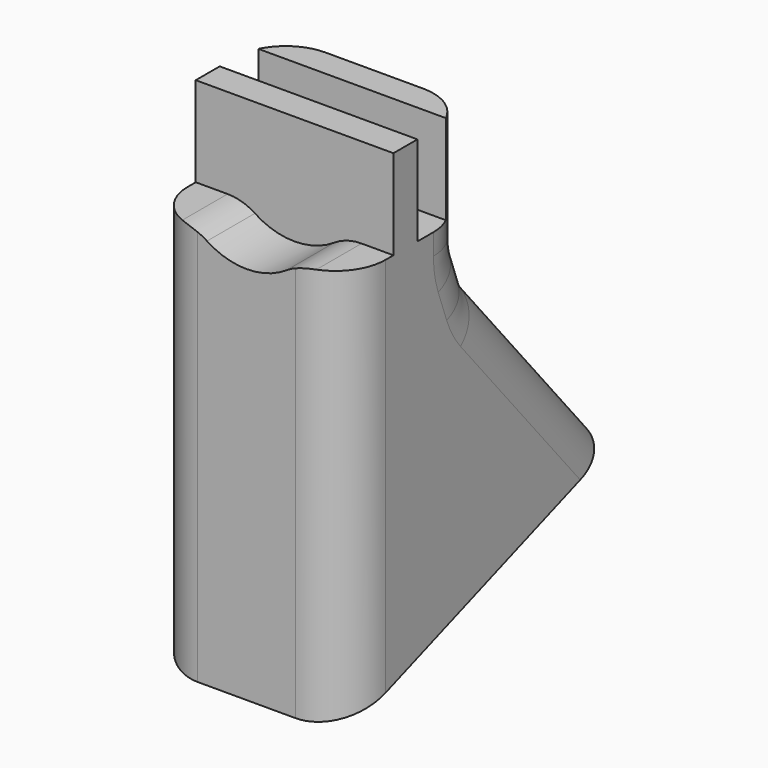
from build123d import *

# Parameters (mm, degrees)
F0_W     = 2.8
F0_H     = 9
F1_DEPTH = 19.8
F3_F1_R  = 5
F3_F2_R  = 5
F4_DEPTH = 6
F5_R     = 5


# Not quite as in the source:
# - a feature of the source that left no trace in its solid (it failed there, or was rolled back) is left out


with BuildPart() as f1:
    # F0 (on Right) → F1 (new body)
    with BuildSketch(Plane.YZ):
        Polygon((0, 9), (0, 0), (3, 0), (3, 2.7590821834), (3, 9), align=None)
        with Locations((8.6, 4.5)):
            Rectangle(F0_W, F0_H)
        Polygon((3, 0), (0, 0), (0, -3), (7.832443736, -3), (5.3151448425, 0), align=None)
        Polygon((7.2, 0), (5.3151448425, 0), (7.832443736, -3), (10, -3), (10, 0), align=None)
        Polygon((0, -3), (0, 0), (-6, 0), (-6, -40), (20.0199263242, -30.5295213202), (11.6604444312, -7.562033581), (7.832443736, -3), align=None)
        Polygon((10, -3), (7.832443736, -3), (11.6604444312, -7.562033581), align=None)
        Polygon((28.3794082171, -27.4869187373), (11.6604444312, -7.562033581), (20.0199263242, -30.5295213202), align=None)
    extrude(amount=F1_DEPTH)

    # F3: fillet of radius 5 on 6 edges, made by hand

    # F3_f1
    f3_f1_edges = [f1.edges().sort_by_distance(p)[0] for p in [
        (9.9, 10, -3),
        (9.9, 11.6604444312, -7.562033581),
    ]]
    fillet(f3_f1_edges, radius=F3_F1_R)

    # F3_f2
    f3_f2_edges = [f1.edges().sort_by_distance(p)[0] for p in [
        (0, -6, -20),
        (19.8, -6, -20),
        (19.8, 20.3032783203, -17.8621619185),
        (0, 20.3032783203, -17.8621619185),
        (0, 11.7272436201, -7.5234670512),
        (19.8, 11.7272436201, -7.5234670512),
    ]]
    fillet(f3_f2_edges, radius=F3_F2_R)

    # F2 (on face) → F4 (cut, through all)
    with BuildSketch(Plane.XZ.offset(6)):
        with BuildLine():
            ThreePointArc((4.9, 0), (9.9, -2), (14.9, 0))
            Line((14.9, 0), (4.9, 0))
        make_face()
    extrude(amount=-F4_DEPTH, mode=Mode.SUBTRACT)

    # F5
    f5_edges = [f1.edges().sort_by_distance(p)[0] for p in [
        (14.9, -2.9995, 0),
        (4.9, -2.9995, 0),
    ]]
    fillet(f5_edges, radius=F5_R)


solid = f1.part
